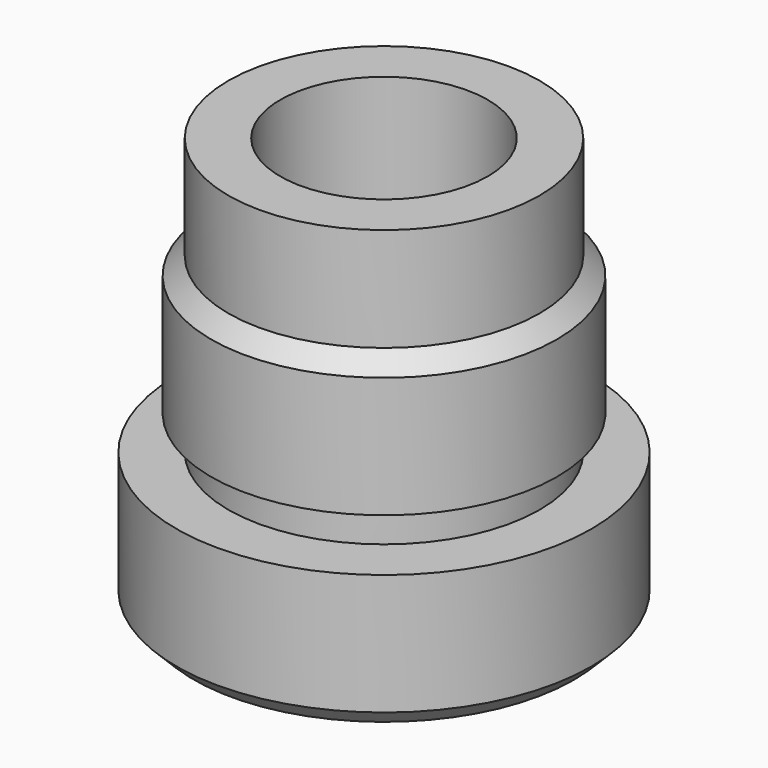
from build123d import *

# Parameters (mm, degrees)
F0_R      = 12
F1_DEPTH  = 8
F2_R      = 10
F3_DEPTH  = 10
F4_R      = 9
F5_DEPTH  = 6
F6_W      = 1
F6_H      = 2
F9_SIZE   = 1
F10_SIZE  = 0.99999
F11_R     = 6
F12_DEPTH = 42.1


# Not quite as in the source:
# - a fillet or chamfer is up to 0.001 mm smaller than in the source, because OpenCascade refuses the exact size


with BuildPart() as f1:
    # F0 (on Top) → F1 (new body)
    with BuildSketch(Plane.XY):
        Circle(F0_R)
    extrude(amount=F1_DEPTH)

    # F2 (on face) → F3 (join)
    with BuildSketch(Plane.XY.offset(8)):
        Circle(F2_R)
    extrude(amount=F3_DEPTH)

    # F4 (on face) → F5 (join)
    with BuildSketch(Plane.XY.offset(18)):
        Circle(F4_R)
    extrude(amount=F5_DEPTH)

    # F6 (on Right) → F8 (revolve, cut)
    with BuildSketch(Plane.YZ):
        with Locations((9.5, 9)):
            Rectangle(F6_W, F6_H)
    revolve(axis=Axis((0, 0, 13.7254064903), (0, 0, 1)), mode=Mode.SUBTRACT)

    # F9
    f9_edges = [f1.edges().sort_by_distance(p)[0] for p in [
        (-12, 0, 0),
    ]]
    chamfer(f9_edges, length=F9_SIZE)

    # F10 (size 1 in the source; OpenCascade refuses exactly that, so slightly less here)
    f10_edges = [f1.edges().sort_by_distance(p)[0] for p in [
        (-10, 0, 18),
    ]]
    chamfer(f10_edges, length=F10_SIZE)

    # F11 (on face) → F12 (cut)
    with BuildSketch(Plane.XY.offset(24)):
        Circle(F11_R)
    extrude(amount=-F12_DEPTH, mode=Mode.SUBTRACT)


solid = f1.part
